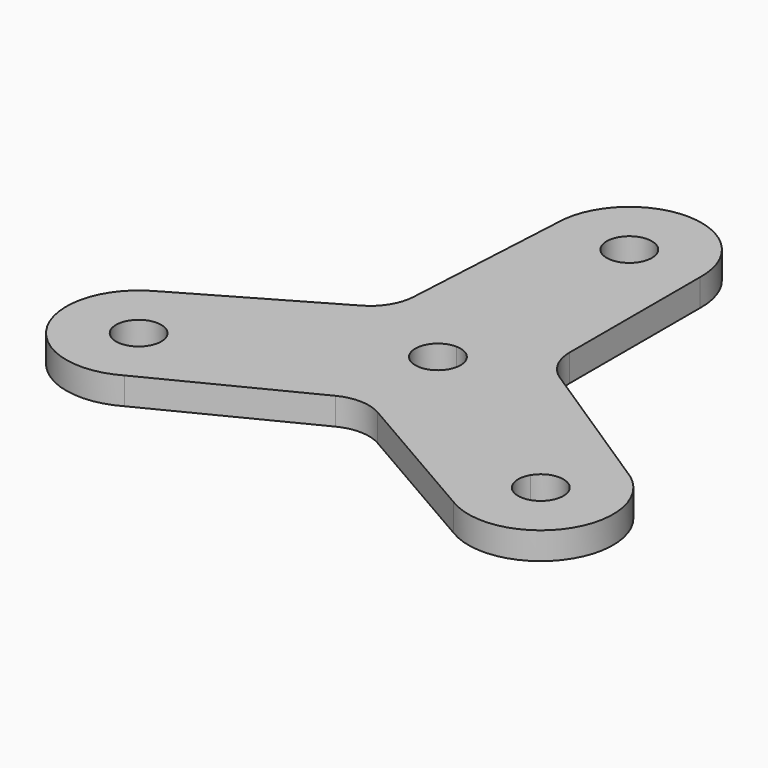
from build123d import *

# Parameters (mm, degrees)
F1_DEPTH = 3


# Not quite as in the source:
# - a feature names something its author has since deleted; it is built from what else it names


with BuildPart() as f1:
    # F0 (on Top) → F1 (new body)
    with BuildSketch(Plane.XY):
        with BuildLine():
            Line((8.3654914829, 7.7478343503), (8.3654914829, 25.7808157751))
            ThreePointArc((8.3654914829, 25.7808157751), (0.4767203504, 33.9966565171), (-7.631576467, 25.9973895632))
            Line((-7.631576467, 25.9973895632), (-8.6528857034, 7.4260866897))
            ThreePointArc((-8.6528857034, 7.4260866897), (-9.3855131516, 5.0826540918), (-11.1453419747, 3.3705145438))
            Line((-11.1453419747, 3.3705145438), (-26.7623619946, -5.6459761686))
            ThreePointArc((-26.7623619946, -5.6459761686), (-29.9331032244, -16.585772745), (-18.951386422, -19.6081302933))
            Line((-18.951386422, -19.6081302933), (-2.3575117339, -11.2069586004))
            ThreePointArc((-2.3575117339, -11.2069586004), (0.038274152, -10.6697162831), (2.400944907, -11.3377029763))
            Line((2.400944907, -11.3377029763), (18.0179649268, -20.3541936886))
            ThreePointArc((18.0179649268, -20.3541936886), (29.0774772891, -17.6302378543), (26.2040573041, -6.6086133521))
            Line((26.2040573041, -6.6086133521), (10.6314918524, 3.5615178285))
            ThreePointArc((10.6314918524, 3.5615178285), (8.9683334147, 5.3677081091), (8.3654914829, 7.7478343503))
        make_face()
        with BuildLine():
            ThreePointArc((-20.451386422, -12.679927063), (-25.3707248656, -13.3098488797), (-20.7688276181, -11.4607318089))
            ThreePointArc((-20.7688276181, -11.4607318089), (-20.5320479783, -12.0500052463), (-20.451386422, -12.679927063))
        make_face(mode=Mode.SUBTRACT)
        with BuildLine():
            ThreePointArc((24.7040573041, -13.5368165824), (21.5399163779, -15.9469860432), (20.0569238399, -12.25626284))
            ThreePointArc((20.0569238399, -12.25626284), (22.8681982302, -11.1266471215), (24.7040573041, -13.5368165824))
        make_face(mode=Mode.SUBTRACT)
        with BuildLine():
            ThreePointArc((-7.9164689421, -4.2812988086), (-7.6979940139, 4.6627125327), (0.127531223, 8.9990963873))
            ThreePointArc((0.127531223, 8.9990963873), (6.4088915191, 6.3187110629), (9, 0))
            ThreePointArc((9, 0), (8.6421794957, -2.5125153857), (7.5971703192, -4.8252464332))
            ThreePointArc((7.5971703192, -4.8252464332), (-0.315369081, -8.9944728774), (-7.9164689421, -4.2812988086))
        make_face(mode=Mode.SUBTRACT)
        with BuildLine():
            ThreePointArc((2.868423533, 25.9973895632), (2.1236210505, 24.217141919), (0.3329981933, 23.4976405667))
            ThreePointArc((0.3329981933, 23.4976405667), (-1.3867739845, 27.7776372074), (2.868423533, 25.9973895632))
        make_face(mode=Mode.SUBTRACT)
        with BuildLine():
            ThreePointArc((0.0354253397, 2.4997489965), (1.7802476442, 1.7551975175), (2.5, 0))
            ThreePointArc((2.5, 0), (2.3734655501, -0.7852778377), (2.0066709741, -1.4910639161))
            Line((2.0066709741, -1.4910639161), (7.5971703192, -4.8252464332))
            ThreePointArc((7.5971703192, -4.8252464332), (8.6421794957, -2.5125153857), (9, 0))
            ThreePointArc((9, 0), (6.4088915191, 6.3187110629), (0.127531223, 8.9990963873))
            Line((0.127531223, 8.9990963873), (0.0354253397, 2.4997489965))
        make_face()
        with BuildLine():
            ThreePointArc((-2.239906233, -1.1103243073), (-2.1149683962, 1.333007383), (0.0354253397, 2.4997489965))
            Line((0.0354253397, 2.4997489965), (0.127531223, 8.9990963873))
            ThreePointArc((0.127531223, 8.9990963873), (-7.6979940139, 4.6627125327), (-7.9164689421, -4.2812988086))
            Line((-7.9164689421, -4.2812988086), (-2.239906233, -1.1103243073))
        make_face()
        with BuildLine():
            Line((7.5971703192, -4.8252464332), (2.0066709741, -1.4910639161))
            ThreePointArc((2.0066709741, -1.4910639161), (-0.2232494881, -2.4900119811), (-2.239906233, -1.1103243073))
            Line((-2.239906233, -1.1103243073), (-7.9164689421, -4.2812988086))
            ThreePointArc((-7.9164689421, -4.2812988086), (-0.315369081, -8.9944728774), (7.5971703192, -4.8252464332))
        make_face()
    extrude(amount=F1_DEPTH)


solid = f1.part
